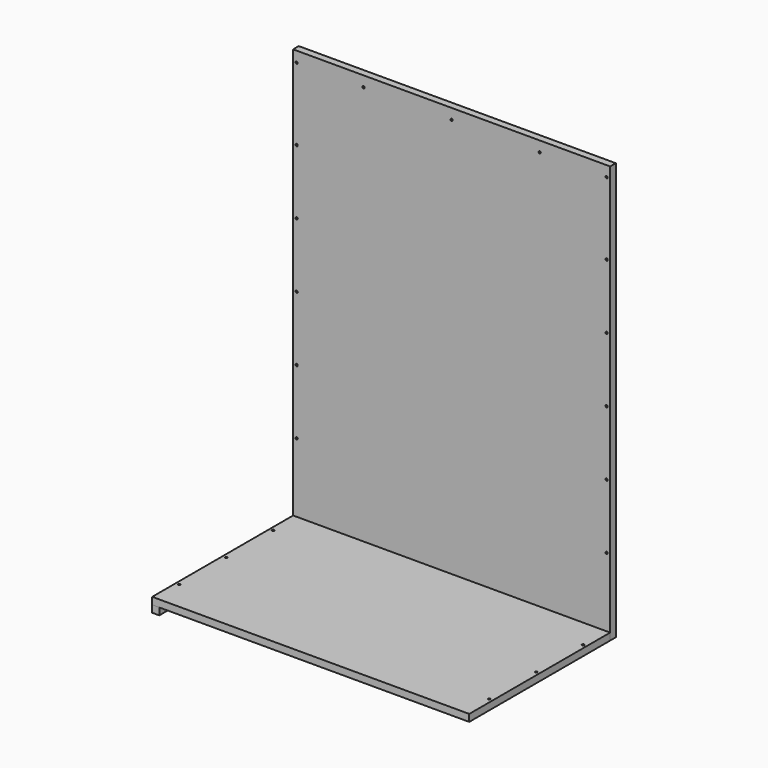
from build123d import *

# Parameters (mm, degrees)
F0_W           = 540
F0_H           = 300
F1_DEPTH       = 12
F3_D           = 3.7973
F3_CSINK_D     = 7.7978
F3_CSINK_ANGLE = 82
F4_W           = 540
F4_H           = 699
F5_DEPTH       = 12
F7_D           = 3.7973
F7_CSINK_D     = 7.7978
F7_CSINK_ANGLE = 82
F8_DEPTH       = 12
F9_W           = 12
F9_H           = 300
F10_DEPTH      = 12


# Not quite as in the source:
# - a pattern or mirror of a feature is missing from the dataset's text; its kind, count and spacing are read off the source's solid


with BuildPart() as f1:
    # F0 (on Top) → F1 (new body)
    with BuildSketch(Plane.XY):
        Rectangle(F0_W, F0_H)
    extrude(amount=F1_DEPTH)

    # F3 (through all)
    with Locations(Plane(origin=(0, 0, 0), x_dir=(1, 0, 0), z_dir=(0, 0, -1))):
        with Locations((-264, -100), (-264, 0), (-264, 100)):
            f3 = CounterSinkHole(F3_D / 2, F3_CSINK_D / 2, counter_sink_angle=F3_CSINK_ANGLE)

    # F3_copies: F3 across plane
    add(f3.mirror(Plane(origin=(0, 0, 0), x_dir=(0, 0, 1), z_dir=(1, 0, 0))), mode=Mode.SUBTRACT)


with BuildPart() as f5:
    # F4 (on face) → F5 (new body)
    with BuildSketch(Plane(origin=(0, 150, 0), x_dir=(-1, 0, 0), z_dir=(0, 1, 0))):
        with Locations((0, 349.5)):
            Rectangle(F4_W, F4_H)
    extrude(amount=F5_DEPTH)

    # F7 (through all)
    with Locations(Plane(origin=(0, 162, 0), x_dir=(-1, 0, 0), z_dir=(0, 1, 0))):
        with Locations((264, 129.5), (264, 239.5), (264, 349.5), (264, 459.5), (264, 569.5), (264, 693), (150, 693), (0, 693), (-150, 693), (-264, 693), (-264, 569.5), (-264, 459.5), (-264, 349.5), (-264, 239.5), (-264, 129.5), (-264, 6), (-150, 6), (0, 6), (150, 6), (264, 6)):
            CounterSinkHole(F7_D / 2, F7_CSINK_D / 2, counter_sink_angle=F7_CSINK_ANGLE)

    # F8 (add): a face of the model
    f8_faces = [f5.faces().sort_by_distance(p)[0] for p in [
        (0, 156, 699),
    ]]
    extrude(f8_faces, amount=F8_DEPTH)


with BuildPart() as f10:
    # F9 (on face) → F10 (new body)
    with BuildSketch(Plane(origin=(0, 0, 0), x_dir=(1, 0, 0), z_dir=(0, 0, -1))):
        with Locations((-264, 0)):
            Rectangle(F9_W, F9_H)
    extrude(amount=F10_DEPTH)


solid = Compound([f1.part, f5.part, f10.part])
